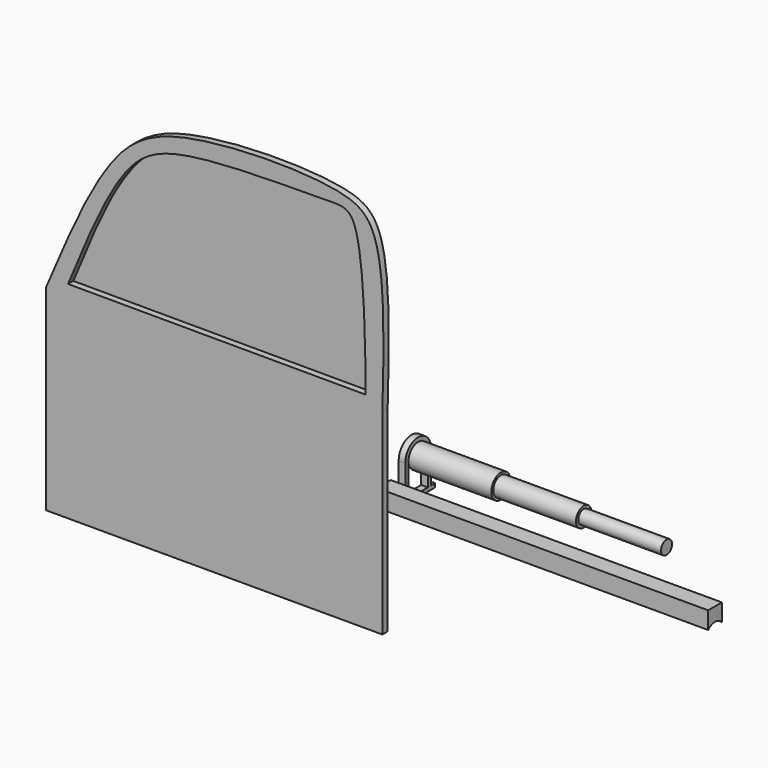
from build123d import *

# Parameters (mm, degrees)
F1_DEPTH  = 2
F3_DEPTH  = 1
F5_DEPTH  = 12.5
F6_R      = 0.6740837688
F6_R_2    = 0.6794872763
F7_DEPTH  = 2
F8_R      = 1.1503813394
F8_R_2    = 1.1532026448
F9_DEPTH  = 1
F15_DEPTH = 100
F16_R     = 3.6496373468
F17_DEPTH = 25
F18_R     = 2.9198473691
F19_DEPTH = 25
F20_R     = 2.0774271532
F21_DEPTH = 25
F23_DEPTH = 2
F24_DEPTH = 2


# Not quite as in the source:
# - a feature names something its author has since deleted; it is built from what else it names


with BuildPart() as f1:
    # F0 (on Front) → F1 (new body)
    with BuildSketch(Plane.XZ):
        with BuildLine():
            Line((-72.9369357123, -81.3669546917), (28.6214776443, -81.3669546917))
            Line((28.6214776443, -81.3669546917), (28.6214776443, -22.0463353619))
            add(Edge.make_bspline(
                [(-72.9369357123, -22.0463353619), (-66.3079296953, -6.3903379982), (-54.8236810491, 20.7324864598), (-33.1368908634, 33.9886563081), (14.1885215953, 34.4693387216), (29.9138992328, 26.3054952003), (29.1285218253, -3.0768949366), (28.6214776443, -22.0463353619)],
                knots=[0, 0, 0, 0, 0.2327586614, 0.4032366747, 0.6349341911, 0.7643114096, 1, 1, 1, 1], degree=3))
            Line((-72.9369357123, -22.0463353619), (-72.9369357123, -81.3669546917))
        make_face()
        with BuildLine():
            Line((23.5529407965, -19.2304815576), (-66.3079296953, -19.0427604541))
            add(Edge.make_bspline(
                [(-66.3079296953, -19.0427604541), (-60.6025988038, -5.2091205775), (-50.8417035049, 18.4579923395), (-32.9418385651, 29.0509048337), (11.2998233245, 28.2534036027), (23.8422582571, 29.4620440208), (23.5609324216, -16.9963213799), (23.5529407965, -19.2304815576)],
                knots=[0, 0, 0, 0, 0.2292277789, 0.3921715308, 0.6301185848, 0.7440435368, 0.9842506716, 0.9842506716, 0.9842506716, 0.9842506716], degree=3))
        make_face(mode=Mode.SUBTRACT)
    extrude(amount=F1_DEPTH)


with BuildPart() as f3:
    # F2 (on face) → F3 (new body)
    with BuildSketch(Plane(origin=(0, 0, 0), x_dir=(-1, 0, 0), z_dir=(0, 1, 0))):
        with BuildLine():
            Line((-23.5529407964, -19.2304815668), (66.3079296953, -19.0427604541))
            add(Edge.make_bspline(
                [(-23.5529407964, -19.2304815668), (-23.269595086, -5.9334404727), (-22.8404862365, 14.5885042855), (-20.184558271, 26.8697861091), (-13.9924322403, 30.0265202781), (31.2151711749, 28.02875343), (44.8400626895, 22.8259909303), (55.9527219343, 6.1579662544), (63.45297845, -12.1512318258), (65.5205113196, -17.1808483014), (66.3079296953, -19.0427604541)],
                knots=[0, 0, 0, 0, 0.1767993283, 0.2727640909, 0.3442462663, 0.5417821056, 0.6587934226, 0.788359659, 0.9213359844, 1, 1, 1, 1], degree=3))
        make_face()
    extrude(amount=F3_DEPTH)


with BuildPart() as f5:
    # F4 (on Right) → F5 (new body, symmetric)
    with BuildSketch(Plane.YZ):
        Polygon((-1.0896978201, -60.7723593712), (-1.0896978201, -72.45323807), (-0.2179905568, -72.45323807), (-0.2179905568, -61.9055777788), (1.0241923155, -61.9055777788), (1.0241923155, -72.45323807), (2.0484484266, -72.45323807), (2.0484484266, -60.7723593712), align=None)
    extrude(amount=F5_DEPTH, both=True)

    # F6 (on face) → F7 (join)
    with BuildSketch(Plane(origin=(0, 2.0484484266, 0), x_dir=(-1, 0, 0), z_dir=(0, 1, 0))):
        with Locations((-10.6959426776, -67.096978426)):
            Circle(F6_R)
        with Locations((10.5811031535, -67.096978426)):
            Circle(F6_R_2)
    extrude(amount=F7_DEPTH)

    # F8 (on face) → F9 (join)
    with BuildSketch(Plane(origin=(0, 4.0484484266, 0), x_dir=(-1, 0, 0), z_dir=(0, 1, 0))):
        with Locations((-10.6959426776, -67.096978426)):
            Circle(F8_R)
        with Locations((10.6070199981, -67.0710653067)):
            Circle(F8_R_2)
    extrude(amount=F9_DEPTH)


with BuildPart() as f11:
    # F10 (on Right) → F11 (revolve)
    with BuildSketch(Plane.YZ):
        with BuildLine():
            Line((2.1344509079, -62.3869039118), (2.0657987334, -62.3869039118))
            Line((2.0657987334, -62.3869039118), (2.0657987334, -67.175835371))
            Line((2.0657987334, -67.175835371), (3.6893903743, -67.175835371))
            Line((3.6893903743, -67.175835371), (3.6893903743, -63.812112902))
            ThreePointArc((3.6893903743, -63.812112902), (3.0686592581, -62.9285025663), (2.1344509079, -62.3869039118))
        make_face()
    revolve(axis=Axis((0, 4.3976157904, -67.175835371), (0, 1, 0)))

    # F12 (on Right) → F13 (revolve)
    with BuildSketch(Plane.YZ):
        with BuildLine():
            Line((3.290206524, -67.100353539), (5.9968891046, -67.100353539))
            ThreePointArc((5.9968891046, -67.100353539), (4.6435478143, -65.7470122487), (3.290206524, -67.100353539))
        make_face()
    revolve(axis=Axis((0, 4.8515796661, -67.100353539), (0, 1, 0)))


with BuildPart() as f15:
    # F14 (on Right) → F15 (new body)
    with BuildSketch(Plane.YZ):
        with BuildLine():
            Line((36.9551664144, -65.4419660568), (31.763907522, -65.4419660568))
            Line((31.763907522, -65.4419660568), (31.763907522, -70.6833247065))
            ThreePointArc((31.763907522, -70.6833247065), (34.3595369682, -69.558063283), (36.9551664144, -70.6833247065))
            Line((36.9551664144, -70.6833247065), (36.9551664144, -65.4419660568))
        make_face()
    extrude(amount=F15_DEPTH)


with BuildPart() as f17:
    # F16 (on Right) → F17 (new body)
    with BuildSketch(Plane.YZ):
        with Locations((47.3034344614, -63.128657639)):
            Circle(F16_R)
    extrude(amount=F17_DEPTH)

    # F18 (on face) → F19 (join)
    with BuildSketch(Plane.YZ.offset(25)):
        with Locations((47.3034344614, -63.128657639)):
            Circle(F18_R)
    extrude(amount=F19_DEPTH)

    # F20 (on face) → F21 (join)
    with BuildSketch(Plane.YZ.offset(50)):
        with Locations((47.3034344614, -63.128657639)):
            Circle(F20_R)
    extrude(amount=F21_DEPTH)


with BuildPart() as f23:
    # F22 (on face) → F23 (new body)
    with BuildSketch(Plane(origin=(0, 0, 0), x_dir=(0, -1, 0), z_dir=(-1, 0, 0))):
        with BuildLine():
            Line((-42.4340814352, -73.0882510543), (-42.4340814352, -63.128657639))
            ThreePointArc((-42.4340814352, -63.128657639), (-47.3034344614, -58.2593046129), (-52.1727874875, -63.128657639))
            Line((-52.1727874875, -63.128657639), (-52.1727874875, -73.0882510543))
            Line((-52.1727874875, -73.0882510543), (-50.9530718081, -73.0882510543))
            Line((-50.9530718081, -73.0882510543), (-50.9530718081, -63.128657639))
            ThreePointArc((-50.9530718081, -63.128657639), (-47.3034344614, -59.4790202923), (-43.6537971146, -63.128657639))
            Line((-43.6537971146, -63.128657639), (-43.6537971146, -73.0882510543))
            Line((-43.6537971146, -73.0882510543), (-42.4340814352, -73.0882510543))
        make_face()
    extrude(amount=F23_DEPTH)


with BuildPart() as f24:
    # F22 (on face) → F24 (new body)
    with BuildSketch(Plane(origin=(0, 0, 0), x_dir=(0, -1, 0), z_dir=(-1, 0, 0))):
        Polygon((-40.837276727, -73.0882510543), (-42.4340814352, -73.0882510543), (-43.6537971146, -73.0882510543), (-50.9530718081, -73.0882510543), (-52.1727874875, -73.0882510543), (-53.7037067115, -73.0882510543), (-53.7037067115, -74.2193683982), (-40.837276727, -74.2193683982), align=None)
    extrude(amount=F24_DEPTH)


solid = Compound([f1.part, f3.part, f5.part, f11.part, f15.part, f17.part, f23.part, f24.part])
